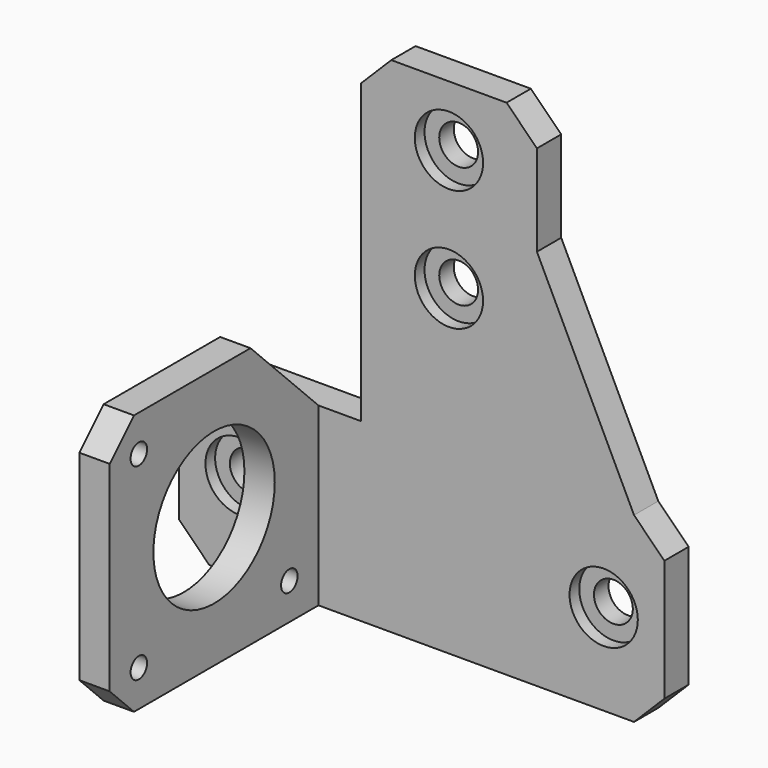
from build123d import *

# Parameters (mm, degrees)
F1_DEPTH       = 5
F2_D           = 6.4
F2_CBORE_D     = 11.25
F2_CBORE_DEPTH = 2
F3_W           = 5
F3_H           = 43
F4_DEPTH       = 43
F6_D           = 3.4
F5_R           = 12.5
F7_DEPTH       = 23.001
F10_DEPTH      = 12
F11_SIZE       = 4.99999


# Not quite as in the source:
# - a fillet or chamfer is up to 0.001 mm smaller than in the source, because OpenCascade refuses the exact size
# - a feature names something its author has since deleted; it is built from what else it names


with BuildPart() as f1:
    # F0 (on Front) → F1 (new body)
    with BuildSketch(Plane.XZ):
        Polygon((0, 29), (0, 0), (80, 0), (80, 30), (75, 30), (59, 63), (59, 83), (30, 83), (30, 43), (18, 43), (18, 29), align=None)
    extrude(amount=-F1_DEPTH)

    # F2 (through all)
    with Locations(Plane.XZ):
        with Locations((10, 14.5), (44.5, 53), (44.5, 73), (70, 15)):
            CounterBoreHole(F2_D / 2, F2_CBORE_D / 2, F2_CBORE_DEPTH)

    # F3 (on face) → F4 (join)
    with BuildSketch(Plane.XZ):
        with Locations((20.5, 21.5)):
            Rectangle(F3_W, F3_H)
    extrude(amount=F4_DEPTH)

    # F6 (through all)
    with Locations(Plane.YZ.offset(23)):
        with Locations((-37, 37), (-6, 6), (-37, 6)):
            Hole(F6_D / 2)

    # F5 (on face) → F7 (cut, through all)
    with BuildSketch(Plane.YZ.offset(23)):
        with Locations((-21.5, 21.5)):
            Circle(F5_R)
    extrude(amount=-F7_DEPTH, mode=Mode.SUBTRACT)

    # F9 (on face) → F10 (cut, through all)
    with BuildSketch(Plane(origin=(18, 0, 0), x_dir=(0, -1, 0), z_dir=(-1, 0, 0))):
        Polygon((14, 43), (-5, 43), (-5, 29), (0, 29), align=None)
    extrude(amount=-F10_DEPTH, mode=Mode.SUBTRACT)

    # F11 (size 5 in the source; OpenCascade refuses exactly that, so slightly less here)
    f11_edges = [f1.edges().sort_by_distance(p)[0] for p in [
        (30, 2.5, 83),
        (59, 2.5, 83),
        (80, 2.5, 30),
        (80, 2.5, 0),
        (20.5, -43, 0),
        (0, 2.5, 0),
        (0, 2.5, 29),
        (20.5, -43, 43),
    ]]
    chamfer(f11_edges, length=F11_SIZE)


solid = f1.part
